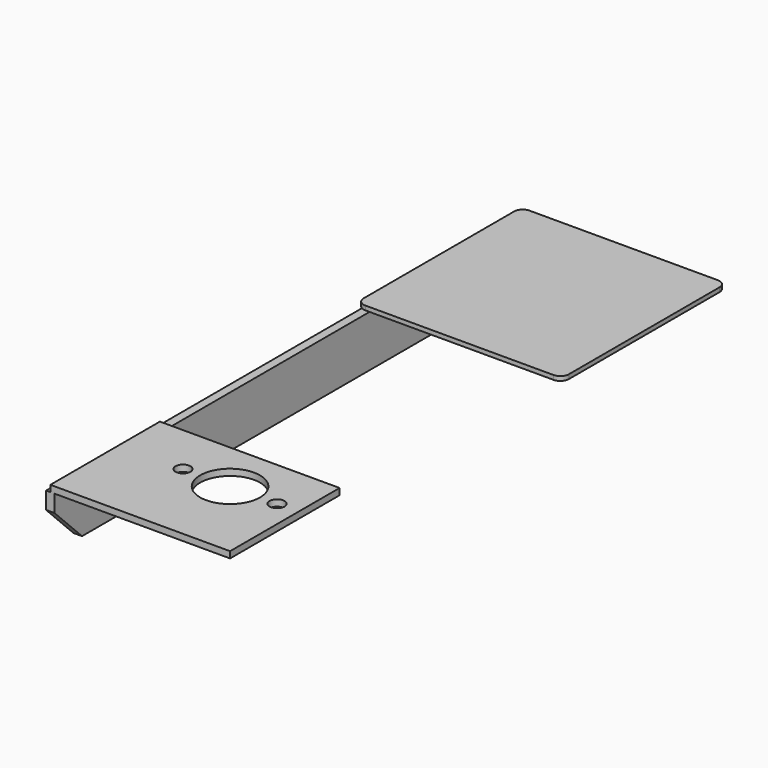
from build123d import *

# Parameters (mm, degrees)
F0_W        = 6.35
F0_H        = 431.8
F1_DEPTH    = 38.1
F2_SIZE     = 25.4
F3_W        = 133.35
F3_H        = 101.6
F4_DEPTH    = 4.7625
F5_R        = 22.225
F5_R_2      = 5.588
F6_DEPTH    = 25.4
F7_W        = 152.4
F7_H        = 152.4
F8_DEPTH    = 3.175
F9_T1_DEPTH = 34.925
F9_T3_DEPTH = 19.05


# Not quite as in the source:
# - a fillet or chamfer that OpenCascade refuses, or shapes differently, is made with other operations: its cross-section is extruded or revolved along the edge and cut away or added


with BuildPart() as f1:
    # F0 (on Top) → F1 (new body)
    with BuildSketch(Plane.XY):
        Rectangle(F0_W, F0_H)
    extrude(amount=-F1_DEPTH)

    # F2
    f2_edges = [f1.edges().sort_by_distance(p)[0] for p in [
        (0, -215.9, -38.1),
        (0, 215.9, -38.1),
    ]]
    chamfer(f2_edges, length=F2_SIZE)

    # F3 (on Top) → F4 (join)
    with BuildSketch(Plane.XY):
        with Locations((66.675, -165.1)):
            Rectangle(F3_W, F3_H)
    extrude(amount=F4_DEPTH)

    # F5 (on face) → F6 (cut)
    with BuildSketch(Plane.XY.offset(4.7625)):
        with Locations((82.55, -152.4)):
            Circle(F5_R)
        with Locations((47.625, -152.4)):
            Circle(F5_R_2)
        with Locations((117.475, -152.4)):
            Circle(F5_R_2)
    extrude(amount=-F6_DEPTH, mode=Mode.SUBTRACT)

    # F7 (on face) → F8 (join)
    with BuildSketch(Plane.XY):
        with Locations((69.85, 152.4)):
            Rectangle(F7_W, F7_H)
    extrude(amount=F8_DEPTH)

    # F9: fillet of radius 6.35 on 4 edges, made by hand

    # F9_s2 → F9_t1 (cut)
    with BuildSketch(Plane.XY.offset(-15.875)):
        with BuildLine():
            ThreePointArc((139.7, 76.2), (144.1901280605, 78.0598719395), (146.05, 82.55))
            Line((146.05, 82.55), (146.05, 76.2))
            Line((146.05, 76.2), (139.7, 76.2))
        make_face()
        with BuildLine():
            ThreePointArc((139.7, 228.6), (144.1901280605, 226.7401280605), (146.05, 222.25))
            Line((146.05, 222.25), (146.05, 228.6))
            Line((146.05, 228.6), (139.7, 228.6))
        make_face()
        with BuildLine():
            ThreePointArc((-6.35, 222.25), (-4.4901280605, 226.7401280605), (0, 228.6))
            Line((0, 228.6), (-6.35, 228.6))
            Line((-6.35, 228.6), (-6.35, 222.25))
        make_face()
    extrude(amount=F9_T1_DEPTH, mode=Mode.SUBTRACT)

    # F9_s4 → F9_t3 (cut)
    with BuildSketch(Plane.XY):
        with BuildLine():
            ThreePointArc((0, 76.2), (-4.4901280605, 78.0598719395), (-6.35, 82.55))
            Line((-6.35, 82.55), (-6.35, 76.2))
            Line((-6.35, 76.2), (0, 76.2))
        make_face()
    extrude(amount=F9_T3_DEPTH, mode=Mode.SUBTRACT)


solid = f1.part
